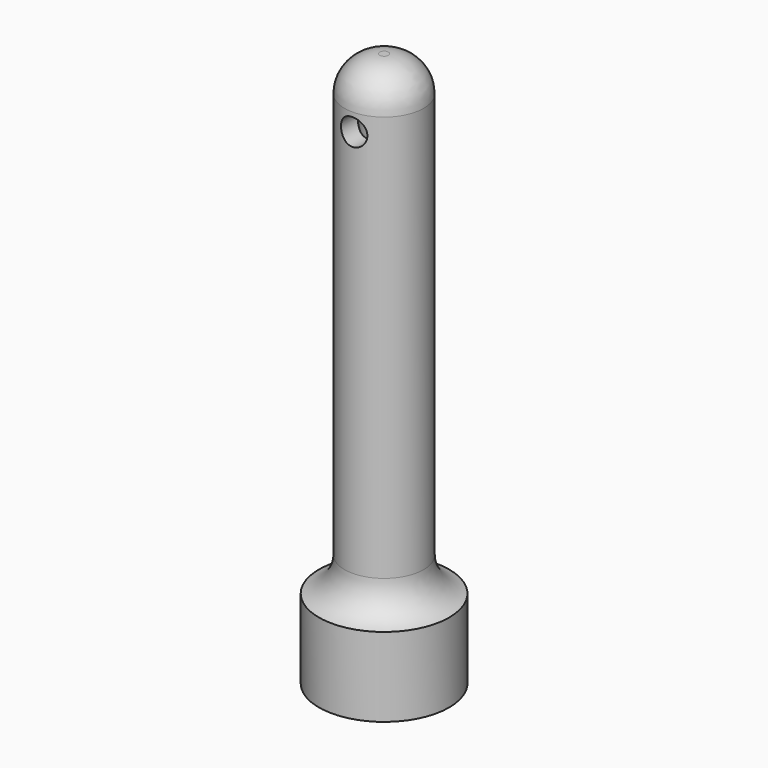
from build123d import *

# Parameters (mm, degrees)
F0_R      = 7.4
F0_R_2    = 2.4
F1_DEPTH  = 3
F2_R      = 7.4
F3_DEPTH  = 3
F4_R      = 4.5
F4_R_2    = 2.4
F5_DEPTH  = 51
F6_DEPTH  = 3
F7_R      = 4.5
F8_DEPTH  = 6
F10_R     = 1.5
F11_DEPTH = 12.5


# Not quite as in the source:
# - a fillet or chamfer that OpenCascade refuses, or shapes differently, is made with other operations: its cross-section is extruded or revolved along the edge and cut away or added


with BuildPart() as f1:
    # F0 (on Top) → F1 (new body)
    with BuildSketch(Plane.XY):
        Circle(F0_R)
        Circle(F0_R_2, mode=Mode.SUBTRACT)
    extrude(amount=F1_DEPTH)

    # F2 (on face) → F3 (join)
    with BuildSketch(Plane.XY.offset(3)):
        Circle(F2_R)
        Polygon((0, 4.1569219382), (3.6, 2.0784609691), (3.6, -2.0784609691), (0, -4.1569219382), (-3.6, -2.0784609691), (-3.6, 2.0784609691), align=None, mode=Mode.SUBTRACT)
    extrude(amount=F3_DEPTH)

    # F4 (on face) → F5 (join)
    with BuildSketch(Plane.XY.offset(6)):
        Circle(F4_R)
        Polygon((-3.6, -2.0784609691), (-3.6, 2.0784609691), (0, 4.1569219382), (3.6, 2.0784609691), (3.6, -2.0784609691), (0, -4.1569219382), align=None, mode=Mode.SUBTRACT)
        Polygon((0, 4.1569219382), (-3.6, 2.0784609691), (-3.6, -2.0784609691), (0, -4.1569219382), (3.6, -2.0784609691), (3.6, 2.0784609691), align=None)
        Circle(F4_R_2, mode=Mode.SUBTRACT)
    extrude(amount=F5_DEPTH)

    # F6 (add): a face of the model
    f6_faces = [f1.faces().sort_by_distance(p)[0] for p in [
        (-7.1906963928, 0, 6),
    ]]
    extrude(f6_faces, amount=F6_DEPTH)

    # F7 (on face) → F8 (join)
    with BuildSketch(Plane.XY.offset(57)):
        Circle(F7_R)
    extrude(amount=F8_DEPTH)

    # F9: fillet of radius 4 on 2 edges, made by hand

    # F9_s1 → F9_t2 (revolve)
    with BuildSketch(Plane.XZ):
        with BuildLine():
            ThreePointArc((7.4, 9), (5.3062561155, 10.4374579888), (4.5, 12.8457769046))
            Line((4.5, 12.8457769046), (4.5, 9))
            Line((4.5, 9), (7.4, 9))
        make_face()
    revolve(axis=Axis((0, 0, 9), (0, 0, 1)))

    # F9_s3 → F9_t4 (revolve, cut)
    with BuildSketch(Plane.XZ):
        with BuildLine():
            ThreePointArc((4.5, 59), (3.3284271247, 61.8284271247), (0.5, 63))
            Line((0.5, 63), (4.5, 63))
            Line((4.5, 63), (4.5, 59))
        make_face()
    revolve(axis=Axis((0, 0, 63), (0, 0, 1)), mode=Mode.SUBTRACT)

    # F10 (on Front) → F11 (cut, symmetric)
    with BuildSketch(Plane.XZ):
        with Locations((0, 57)):
            Circle(F10_R)
    extrude(amount=F11_DEPTH, both=True, mode=Mode.SUBTRACT)


solid = f1.part
